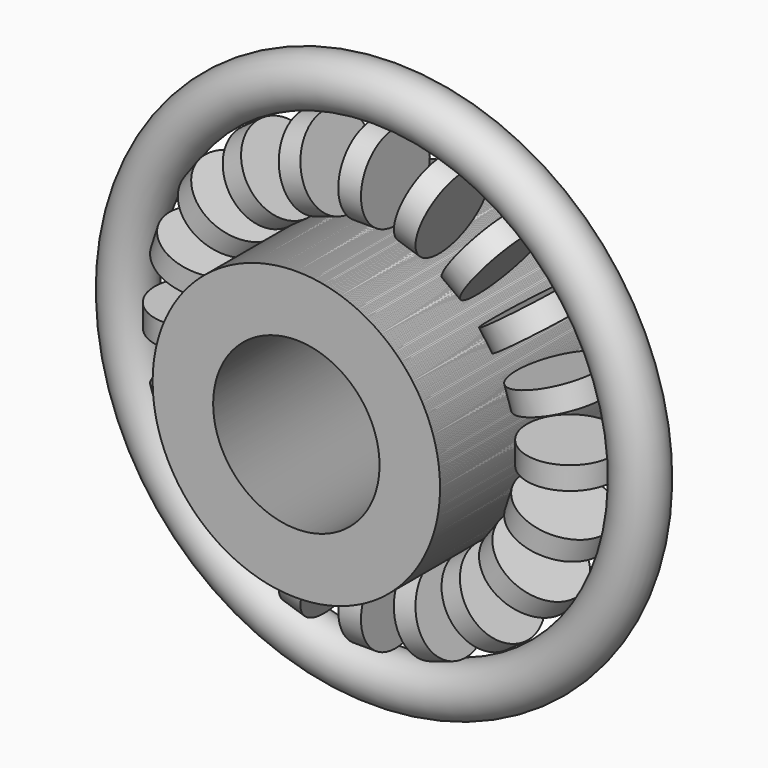
from build123d import *

# Parameters (mm, degrees)
F0_W          = 59.3424290419
F0_H          = 15.9427374601
F2_R          = 11.3579627447
F3_DEPTH      = 3
F3_DEPTH_BACK = 3
F5_COUNT      = 20
F7_R          = 6.6444584542
F9_T          = -1.5


with BuildPart() as f1:
    # F0 (on Right) → F1 (revolve)
    with BuildSketch(Plane.YZ):
        with Locations((0.738106668, 29.9664661288)):
            Rectangle(F0_W, F0_H)
    revolve(axis=Axis((0, 0.8119121194, 0), (0, 1, 0)))

    # F2 (on Right) → F3 (join, two sides)
    with BuildSketch(Plane.YZ) as f3_sk:
        with Locations((0, 49.1567999125)):
            Circle(F2_R)
    extrude(amount=F3_DEPTH)
    extrude(f3_sk.sketch, amount=-F3_DEPTH_BACK)


with BuildPart() as f5_1:
    # F5: instance of F1
    add(f1.part.rotate(Axis((0, 0, 0), (0, -1, 0)), 1 * 360 / F5_COUNT))


with BuildPart() as f5_2:
    # F5: instance of F1
    add(f1.part.rotate(Axis((0, 0, 0), (0, -1, 0)), 2 * 360 / F5_COUNT))


with BuildPart() as f5_3:
    # F5: instance of F1
    add(f1.part.rotate(Axis((0, 0, 0), (0, -1, 0)), 3 * 360 / F5_COUNT))


with BuildPart() as f5_4:
    # F5: instance of F1
    add(f1.part.rotate(Axis((0, 0, 0), (0, -1, 0)), 4 * 360 / F5_COUNT))


with BuildPart() as f5_5:
    # F5: instance of F1
    add(f1.part.rotate(Axis((0, 0, 0), (0, -1, 0)), 5 * 360 / F5_COUNT))


with BuildPart() as f5_6:
    # F5: instance of F1
    add(f1.part.rotate(Axis((0, 0, 0), (0, -1, 0)), 6 * 360 / F5_COUNT))


with BuildPart() as f5_7:
    # F5: instance of F1
    add(f1.part.rotate(Axis((0, 0, 0), (0, -1, 0)), 7 * 360 / F5_COUNT))


with BuildPart() as f5_8:
    # F5: instance of F1
    add(f1.part.rotate(Axis((0, 0, 0), (0, -1, 0)), 8 * 360 / F5_COUNT))


with BuildPart() as f5_9:
    # F5: instance of F1
    add(f1.part.rotate(Axis((0, 0, 0), (0, -1, 0)), 9 * 360 / F5_COUNT))


with BuildPart() as f5_10:
    # F5: instance of F1
    add(f1.part.rotate(Axis((0, 0, 0), (0, -1, 0)), 10 * 360 / F5_COUNT))


with BuildPart() as f5_11:
    # F5: instance of F1
    add(f1.part.rotate(Axis((0, 0, 0), (0, -1, 0)), 11 * 360 / F5_COUNT))


with BuildPart() as f5_12:
    # F5: instance of F1
    add(f1.part.rotate(Axis((0, 0, 0), (0, -1, 0)), 12 * 360 / F5_COUNT))


with BuildPart() as f5_13:
    # F5: instance of F1
    add(f1.part.rotate(Axis((0, 0, 0), (0, -1, 0)), 13 * 360 / F5_COUNT))


with BuildPart() as f5_14:
    # F5: instance of F1
    add(f1.part.rotate(Axis((0, 0, 0), (0, -1, 0)), 14 * 360 / F5_COUNT))


with BuildPart() as f5_15:
    # F5: instance of F1
    add(f1.part.rotate(Axis((0, 0, 0), (0, -1, 0)), 15 * 360 / F5_COUNT))


with BuildPart() as f5_16:
    # F5: instance of F1
    add(f1.part.rotate(Axis((0, 0, 0), (0, -1, 0)), 16 * 360 / F5_COUNT))


with BuildPart() as f5_17:
    # F5: instance of F1
    add(f1.part.rotate(Axis((0, 0, 0), (0, -1, 0)), 17 * 360 / F5_COUNT))


with BuildPart() as f5_18:
    # F5: instance of F1
    add(f1.part.rotate(Axis((0, 0, 0), (0, -1, 0)), 18 * 360 / F5_COUNT))


with BuildPart() as f5_19:
    # F5: instance of F1
    add(f1.part.rotate(Axis((0, 0, 0), (0, -1, 0)), 19 * 360 / F5_COUNT))


with BuildPart() as f8:
    # F7 (on Right) → F8 (revolve)
    with BuildSketch(Plane.YZ):
        with Locations((0, 67.6090493798)):
            Circle(F7_R)
    revolve(axis=Axis((0, 5.0928369164, 0), (0, 1, 0)))

    # F9 (hollow: no face is removed)
    offset(amount=F9_T, mode=Mode.SUBTRACT)


solid = Compound([f1.part, f5_1.part, f5_2.part, f5_3.part, f5_4.part, f5_5.part, f5_6.part, f5_7.part, f5_8.part, f5_9.part, f5_10.part, f5_11.part, f5_12.part, f5_13.part, f5_14.part, f5_15.part, f5_16.part, f5_17.part, f5_18.part, f5_19.part, f8.part])
